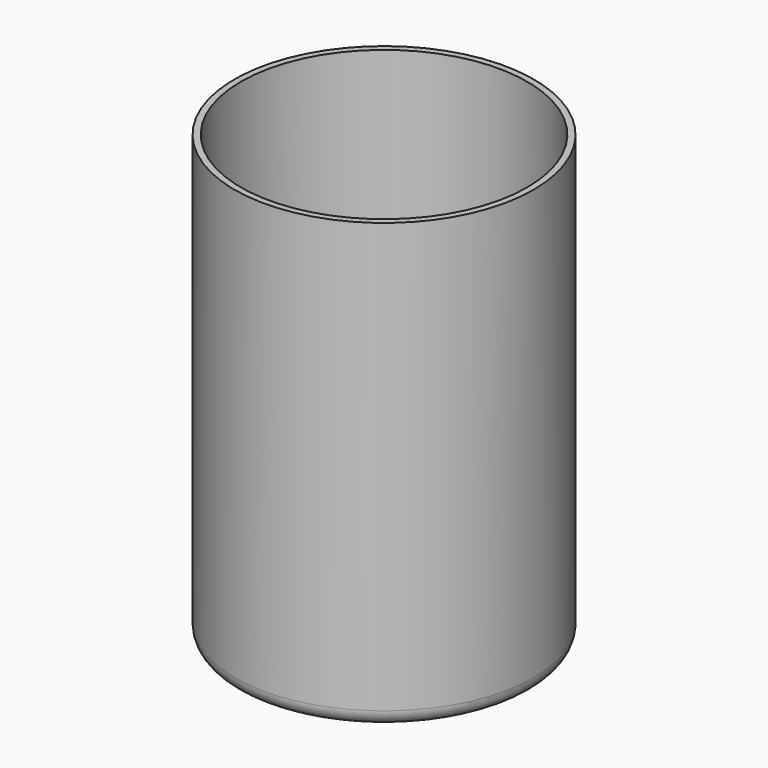
from build123d import *

# Parameters (mm, degrees)
F0_R     = 45.5439388368
F1_DEPTH = 139.7
F2_T     = 2.032
F5_D     = 6.35
F6_D     = 6.35
F7_D     = 6.35


# Not quite as in the source:
# - a fillet or chamfer that OpenCascade refuses, or shapes differently, is made with other operations: its cross-section is extruded or revolved along the edge and cut away or added


with BuildPart() as f1:
    # F0 (on Top) → F1 (new body)
    with BuildSketch(Plane.XY):
        Circle(F0_R)
    extrude(amount=-F1_DEPTH)

    # F2
    f2_openings = [f1.faces().sort_by_distance(p)[0] for p in [
        (0, 0, 0),
    ]]
    offset(amount=F2_T, openings=f2_openings, kind=Kind.INTERSECTION)

    # F3: fillet of radius 5.08 on 1 edges, made by hand

    # F3_s1 → F3_t2 (revolve, cut)
    with BuildSketch(Plane.XZ):
        with BuildLine():
            ThreePointArc((47.5759388368, -136.652), (46.0880412852, -140.2441024484), (42.4959388368, -141.732))
            Line((42.4959388368, -141.732), (47.5759388368, -141.732))
            Line((47.5759388368, -141.732), (47.5759388368, -136.652))
        make_face()
    revolve(axis=Axis((0, 0, -141.732), (0, 0, 1)), mode=Mode.SUBTRACT)

    # F5 (through all)
    with Locations(Plane(origin=(0, 0, -141.732), x_dir=(1, 0, 0), z_dir=(0, 0, -1))):
        with Locations((-8.5982947547, 6.4940573648), (-8.1184855662, 21.5309672058), (-14.8330600932, 26.4003239572), (-7.0802457631, 36.3871436566), (-26.5492741019, 24.3456372991), (-23.826636374, 16.2156112492), (-21.2479694184, 6.4940573648), (-33.2053042948, 4.1952142492)):
            Hole(F5_D / 2)

    # F6 (through all)
    with Locations(Plane(origin=(0, 0, -141.732), x_dir=(1, 0, 0), z_dir=(0, 0, -1))):
        with Locations((8.5982947547, 6.4940573648), (21.2479694184, 6.4940573648), (33.2053042948, 4.1952142492), (8.1184855662, 21.5309672058), (14.8330600932, 26.4003239572), (7.0802457631, 36.3871436566), (23.826636374, 16.2156112492), (26.5492741019, 24.3456372991)):
            Hole(F6_D / 2)

    # F7 (through all)
    with Locations(Plane(origin=(0, 0, -141.732), x_dir=(1, 0, 0), z_dir=(0, 0, -1))):
        with Locations((-33.2053042948, -4.1952142492), (-8.5982947547, -6.4940573648), (-21.2479694184, -6.4940573648), (-8.1184855662, -21.5309672058), (-14.8330600932, -26.4003239572), (-7.0802457631, -36.3871436566), (-26.5492741019, -24.3456372991), (-23.826636374, -16.2156112492), (8.5982947547, -6.4940573648), (33.2053042948, -4.1952142492), (21.2479694184, -6.4940573648), (23.826636374, -16.2156112492), (26.5492741019, -24.3456372991), (14.8330600932, -26.4003239572), (8.1184855662, -21.5309672058), (7.0802457631, -36.3871436566)):
            Hole(F7_D / 2)


solid = f1.part
